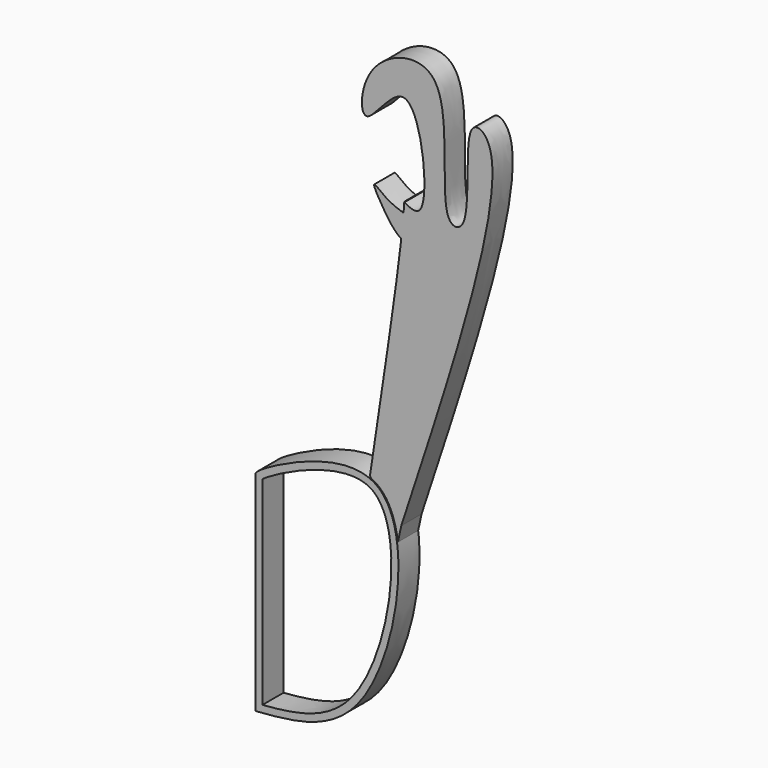
from build123d import *

# Parameters (mm, degrees)
F1_DEPTH = 19.812
F3_DEPTH = 19.05


# Not quite as in the source:
# - ends of sketch curves that miss each other by under 0.0002 mm in the source are joined
# - the dataset's text gives a spline's control points without its knots; the knots are read off the source's solid


with BuildPart() as f1:
    # F0 (on Front) → F1 (new body)
    with BuildSketch(Plane.XZ):
        with BuildLine():
            add(Edge.make_bspline(
                [(0, 76.5141323209), (0.7433221206, 77.4727347098), (4.2208074345, 81.9573661192), (129.2322701811, 146.527090065), (98.7390819728, -73.1223504124), (30.127405598, -78.4310926545), (0, -80.7621628046)],
                knots=[0, 0, 0, 0, 0.0760777767, 0.3559148097, 0.7171820192, 1, 1, 1, 1], degree=3))
            Line((0, 76.5141323209), (0, -80.7621628046))
        make_face()
        with BuildLine():
            Line((5.3339975098, -74.9916417322), (5.3339975098, 74.4165874588))
            add(Edge.make_bspline(
                [(5.3339975098, 74.4165874588), (5.3470249016, 74.4273445717), (5.6066241481, 74.6400712104), (6.2943893902, 75.1672938136), (7.9436076535, 76.2800916687), (10.3345031542, 77.7586623382), (13.3480605318, 79.5037600845), (16.9097897451, 81.4487427766), (20.9461603408, 83.5284163342), (26.8684700965, 86.3983964826), (35.1129418117, 90.0148169838), (45.802240754, 93.9184695492), (56.7214553983, 96.9133785696), (65.5135589605, 98.2734182055), (72.0392493825, 98.4881698363), (76.5962624569, 98.1798640517), (80.0486810116, 97.5151806004), (82.5767801734, 96.7361592063), (84.3529852227, 96.0281556728), (86.0108043388, 95.194183623), (87.5480188561, 94.2333202416), (89.0113238405, 93.1149119401), (90.8695346792, 91.4106340766), (93.0263860403, 88.8699280435), (95.3377948251, 85.1583031161), (97.3442614407, 80.8109493537), (99.5815704989, 74.2327874747), (101.5156534269, 64.694911683), (102.4311923361, 51.6623687521), (101.9948122772, 37.5495193287), (100.2904737, 22.8426813505), (97.4178971715, 8.0158800552), (93.4860440929, -6.4629949473), (89.4247018298, -17.8496950984), (85.7706469294, -26.3161297311), (82.8463610758, -32.2850243572), (80.2737801468, -36.8912798472), (78.1458469019, -40.3263748531), (75.9777410144, -43.5817156034), (73.1863258727, -47.3217394843), (69.7108276375, -51.327530526), (66.1164687408, -54.8859598532), (61.1694589608, -59.0833016592), (54.6993512581, -63.3926734884), (46.4741355911, -67.3179154699), (37.7961742848, -70.2117000663), (28.7032965731, -72.2698208225), (17.9276416684, -73.8889650128), (10.0288493535, -74.6094872809), (5.3339975098, -74.9916417322)],
                knots=[0.0460323986, 0.0460323986, 0.0460323986, 0.0460323986, 0.046875, 0.0625, 0.078125, 0.09375, 0.109375, 0.125, 0.140625, 0.15625, 0.1875, 0.21875, 0.25, 0.28125, 0.296875, 0.3125, 0.328125, 0.3359375, 0.34375, 0.3515625, 0.359375, 0.3671875, 0.375, 0.390625, 0.40625, 0.421875, 0.4375, 0.46875, 0.5, 0.53125, 0.5625, 0.59375, 0.625, 0.65625, 0.671875, 0.6875, 0.703125, 0.7109375, 0.71875, 0.734375, 0.75, 0.765625, 0.78125, 0.8125, 0.84375, 0.875, 0.90625, 0.9375, 0.9819491349, 0.9819491349, 0.9819491349, 0.9819491349], degree=3))
        make_face(mode=Mode.SUBTRACT)
    extrude(amount=F1_DEPTH)


with BuildPart() as f3:
    # F2 (on Front) → F3 (new body)
    with BuildSketch(Plane.XZ):
        with BuildLine():
            add(Edge.make_bspline(
                [(85.5253111922, 102.321335835), (95.5141012767, 168.1775650877), (105.2523692318, 232.7410673995), (109.0698167682, 266.7523622513)],
                knots=[0.0293406646, 0.0293406646, 0.0293406646, 0.0293406646, 0.6934349742, 0.6934349742, 0.6934349742, 0.6934349742], degree=3))
            Line((85.5253111922, 102.321335835), (106.4144303967, 64.7480017278))
            Line((106.4144303967, 64.7480017278), (109.0698167682, 77.0077928901))
            add(Edge.make_bspline(
                [(111.3325704752, 291.6428361883), (116.2183880723, 289.1535381797), (132.6926214708, 280.7600041238), (120.1969146902, 395.3633975273), (77.2067683812, 318.716053131), (78.2843117922, 380.9538231452), (155.710687236, 404.0243883285), (133.4430208753, 286.9006741327), (164.5491628787, 286.7605963446), (152.7662718006, 367.33728622), (197.7988355016, 345.6615215019), (149.1065563473, 198.2310355557), (109.0698167682, 77.0077928901)],
                knots=[0, 0, 0, 0, 0.0493719341, 0.1664746483, 0.249355046, 0.3278511656, 0.4238427426, 0.5565470026, 0.6010421731, 0.7144247599, 0.7651886148, 1, 1, 1, 1], degree=3))
            Line((111.3325704752, 291.6428361883), (111.3325704752, 292.1324876105))
            add(Edge.make_bspline(
                [(110.7902975697, 284.4974967904), (111.0064640685, 287.2252080961), (111.1811108001, 289.738671975), (111.3325704752, 292.1324876105)],
                knots=[0.8305777158, 0.8305777158, 0.8305777158, 0.8305777158, 0.9053847275, 0.9053847275, 0.9053847275, 0.9053847275], degree=3))
            add(Edge.make_bspline(
                [(109.0698167682, 266.7523622513), (109.8581614557, 273.776066797), (110.3940022811, 279.4968184009), (110.7902975697, 284.4974967904)],
                knots=[0.6934349742, 0.6934349742, 0.6934349742, 0.6934349742, 0.8305777158, 0.8305777158, 0.8305777158, 0.8305777158], degree=3))
        make_face()
        with BuildLine():
            add(Edge.make_bspline(
                [(109.0698167682, 266.7523622513), (106.8265668797, 268.3414508562), (101.2060018924, 272.3214832246), (82.8849286861, 303.0184006742), (98.0258633232, 288.657863336), (106.2743468489, 285.9837473117), (110.7902975697, 284.4974967904)],
                knots=[0, 0, 0, 0, 0.2166162443, 0.5418835978, 0.7466420799, 1, 1, 1, 1], degree=3))
            add(Edge.make_bspline(
                [(109.0698167682, 266.7523622513), (109.8581614557, 273.776066797), (110.3940022811, 279.4968184009), (110.7902975697, 284.4974967904)],
                knots=[0.6934349742, 0.6934349742, 0.6934349742, 0.6934349742, 0.8305777158, 0.8305777158, 0.8305777158, 0.8305777158], degree=3))
        make_face()
    extrude(amount=F3_DEPTH)


solid = Compound([f1.part, f3.part])
